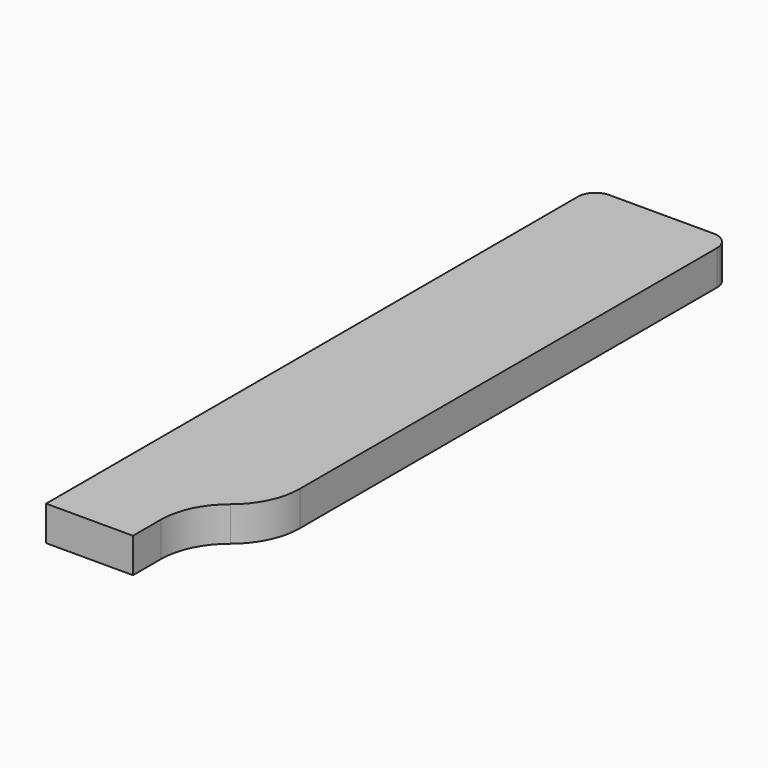
from build123d import *

# Parameters (mm, degrees)
F1_DEPTH = 25.4


# Not quite as in the source:
# - a feature of the source that left no trace in its solid (it failed there, or was rolled back) is left out


with BuildPart() as f1:
    # F0 (on Top) → F1 (new body)
    with BuildSketch(Plane.XY):
        with BuildLine():
            Line((0, 485.775), (0, 0))
            Line((0, 0), (63.5, 0))
            Line((63.5, 0), (63.5, 25.4))
            ThreePointArc((63.5, 25.4), (68.5094988016, 47.3970452561), (82.55, 65.0557372898))
            ThreePointArc((82.55, 65.0557372898), (96.5905011984, 82.7144293235), (101.6, 104.7114745797))
            Line((101.6, 104.7114745797), (101.6, 485.775))
            ThreePointArc((101.6, 485.775), (97.8802561211, 494.7552561211), (88.9, 498.475))
            Line((88.9, 498.475), (12.7, 498.475))
            ThreePointArc((12.7, 498.475), (3.7197438789, 494.7552561211), (0, 485.775))
        make_face()
    extrude(amount=F1_DEPTH)


solid = f1.part
